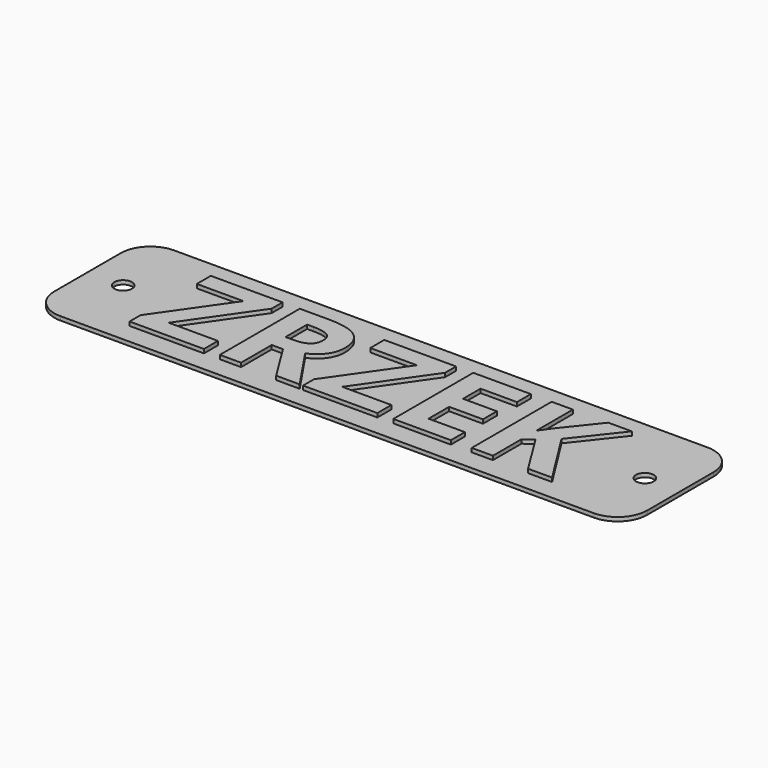
from build123d import *

# Parameters (mm, degrees)
F0_R         = 1.5
F0_TEXT_SIZE = 23.6111111111
F1_DEPTH     = 0.66
F2_DEPTH     = 1.32


# Not quite as in the source:
# - Text() gives the source's letters only with a copy of the font that has no kerning and outlines rounded to 1/6400 em; it was checked with that copy


with BuildPart() as f1:
    # F0 (on Top) → F1 (new body)
    with BuildSketch(Plane.XY):
        with BuildLine():
            Line((45, 12), (-45, 12))
            ThreePointArc((-45, 12), (-48.5355339059, 10.5355339059), (-50, 7))
            Line((-50, 7), (-50, -7))
            ThreePointArc((-50, -7), (-48.5355339059, -10.5355339059), (-45, -12))
            Line((-45, -12), (45, -12))
            ThreePointArc((45, -12), (48.5355339059, -10.5355339059), (50, -7))
            Line((50, -7), (50, 7))
            ThreePointArc((50, 7), (48.5355339059, 10.5355339059), (45, 12))
        make_face()
        Polygon((-23.57421875, -5.5486111111), (-23.57421875, -8.5), (-36.1176215278, -8.5), (-36.1176215278, -6.1831597222), (-28.0345052083, 5.4047309028), (-35.8962673611, 5.4047309028), (-35.8962673611, 8.3561197917), (-23.7918836806, 8.3561197917), (-23.7918836806, 6.0503472222), (-31.8639322917, -5.5486111111), align=None, mode=Mode.SUBTRACT)
        with BuildLine():
            Line((-15.4136284722, -2.0327690972), (-17.3135850694, -2.0327690972))
            Line((-17.3135850694, -2.0327690972), (-17.3135850694, -8.5))
            Line((-17.3135850694, -8.5), (-20.8884548611, -8.5))
            Line((-20.8884548611, -8.5), (-20.8884548611, 8.3561197917))
            Line((-20.8884548611, 8.3561197917), (-15.9780815972, 8.3561197917))
            add(Edge.make_bspline(
                [(-15.9780815972, 8.3561197917), (-12.5397135417, 8.3561197917), (-10.8924696181, 7.10546875)],
                knots=[0, 0, 0, 1, 1, 1], degree=2))
            add(Edge.make_bspline(
                [(-10.8924696181, 7.10546875), (-9.2452256944, 5.8548177083), (-9.2452256944, 3.3055555556)],
                knots=[0, 0, 0, 1, 1, 1], degree=2))
            add(Edge.make_bspline(
                [(-9.2452256944, 3.3055555556), (-9.2452256944, 1.8187934028), (-10.0623914931, 0.6603732639)],
                knots=[0, 0, 0, 1, 1, 1], degree=2))
            add(Edge.make_bspline(
                [(-10.0623914931, 0.6603732639), (-10.8795572917, -0.498046875), (-12.3810763889, -1.1547309028)],
                knots=[0, 0, 0, 1, 1, 1], degree=2))
            add(Edge.make_bspline(
                [(-12.3810763889, -1.1547309028), (-8.5737847222, -6.83984375), (-7.4227430556, -8.5)],
                knots=[0, 0, 0, 1, 1, 1], degree=2))
            Line((-7.4227430556, -8.5), (-11.388671875, -8.5))
            Line((-11.388671875, -8.5), (-15.4136284722, -2.0327690972))
        make_face(mode=Mode.SUBTRACT)
        Polygon((5.6851128472, -5.5486111111), (5.6851128472, -8.5), (-6.8582899306, -8.5), (-6.8582899306, -6.1831597222), (1.2248263889, 5.4047309028), (-6.6369357639, 5.4047309028), (-6.6369357639, 8.3561197917), (5.4674479167, 8.3561197917), (5.4674479167, 6.0503472222), (-2.6046006944, -5.5486111111), align=None, mode=Mode.SUBTRACT)
        Polygon((18.0772569444, -5.5486111111), (18.0772569444, -8.5), (8.3708767361, -8.5), (8.3708767361, 8.3561197917), (18.0772569444, 8.3561197917), (18.0772569444, 5.4268663194), (11.9457465278, 5.4268663194), (11.9457465278, 1.7265625), (17.6529947917, 1.7265625), (17.6529947917, -1.2026909722), (11.9457465278, -1.2026909722), (11.9457465278, -5.5486111111), align=None, mode=Mode.SUBTRACT)
        Polygon((29.2261284722, 0.896484375), (35.1510416667, -8.5), (31.0928819444, -8.5), (26.6768663194, -1.3982204861), (25.16796875, -2.4828559028), (25.16796875, -8.5), (21.5930989583, -8.5), (21.5930989583, 8.3561197917), (25.16796875, 8.3561197917), (25.16796875, 0.6419270833), (26.5735677083, 2.6267361111), (31.1408420139, 8.3561197917), (35.1067708333, 8.3561197917), align=None, mode=Mode.SUBTRACT)
        with Locations((-44, 0)):
            Circle(F0_R, mode=Mode.SUBTRACT)
        with Locations((44, 0)):
            Circle(F0_R, mode=Mode.SUBTRACT)
        with Locations((-36.6820746528, -8.5)):
            Text('ZRZEK', F0_TEXT_SIZE, font='Open Sans', font_style=FontStyle.BOLD, text_align=(TextAlign.LEFT, TextAlign.BOTTOM))
        with BuildLine():
            Line((-17.3135850694, 5.4268663194), (-17.3135850694, 0.8743489583))
            Line((-17.3135850694, 0.8743489583), (-16.1625434028, 0.8743489583))
            add(Edge.make_bspline(
                [(-16.1625434028, 0.8743489583), (-14.4654947917, 0.8743489583), (-13.6593967014, 1.4388020833)],
                knots=[0, 0, 0, 1, 1, 1], degree=2))
            add(Edge.make_bspline(
                [(-13.6593967014, 1.4388020833), (-12.8532986111, 2.0032552083), (-12.8532986111, 3.2133246528)],
                knots=[0, 0, 0, 1, 1, 1], degree=2))
            add(Edge.make_bspline(
                [(-12.8532986111, 3.2133246528), (-12.8532986111, 4.4123263889), (-13.6778428819, 4.9195963542)],
                knots=[0, 0, 0, 1, 1, 1], degree=2))
            add(Edge.make_bspline(
                [(-13.6778428819, 4.9195963542), (-14.5023871528, 5.4268663194), (-16.2289496528, 5.4268663194)],
                knots=[0, 0, 0, 1, 1, 1], degree=2))
            Line((-16.2289496528, 5.4268663194), (-17.3135850694, 5.4268663194))
        make_face()
    extrude(amount=F1_DEPTH)

    # F0 (on Top) → F2 (join)
    with BuildSketch(Plane.XY):
        with Locations((-36.6820746528, -8.5)):
            Text('ZRZEK', F0_TEXT_SIZE, font='Open Sans', font_style=FontStyle.BOLD, text_align=(TextAlign.LEFT, TextAlign.BOTTOM))
    extrude(amount=F2_DEPTH)


solid = f1.part
